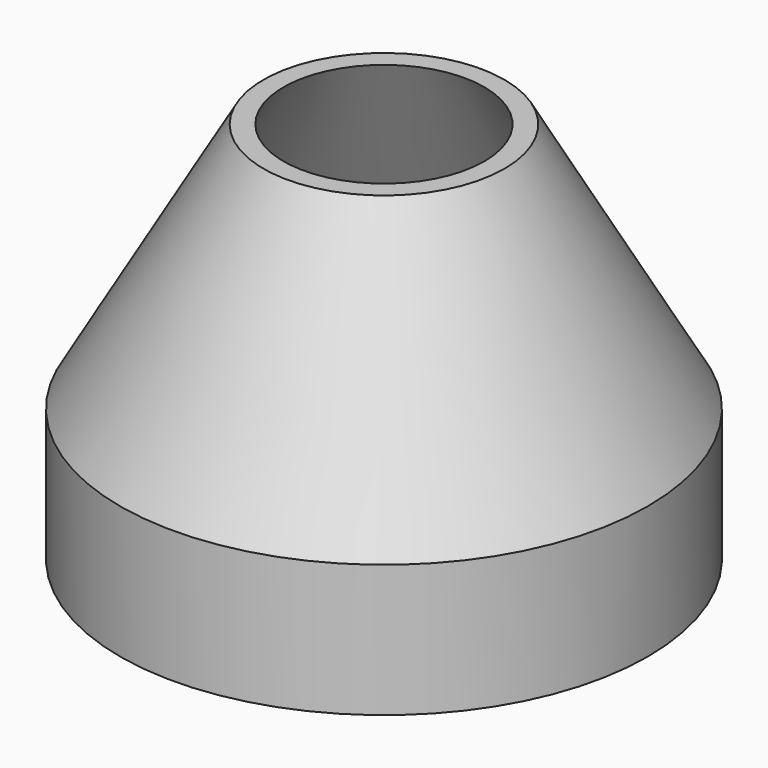
from build123d import *


# Not quite as in the source:
# - a feature names something its author has since deleted; it is built from what else it names


with BuildPart() as f1:
    # F0 (on Front) → F1 (revolve)
    with BuildSketch(Plane.XZ):
        Polygon((12, 63.5863808764), (10, 63.5863808764), (24.28, 38.5863808764), (24.28, 25.4715627463), (26.28, 25.4715627463), (26.28, 38.6495627463), align=None)
    revolve(axis=Axis((0, 0, 35.6375661366), (0, 0, -1)))


solid = f1.part
